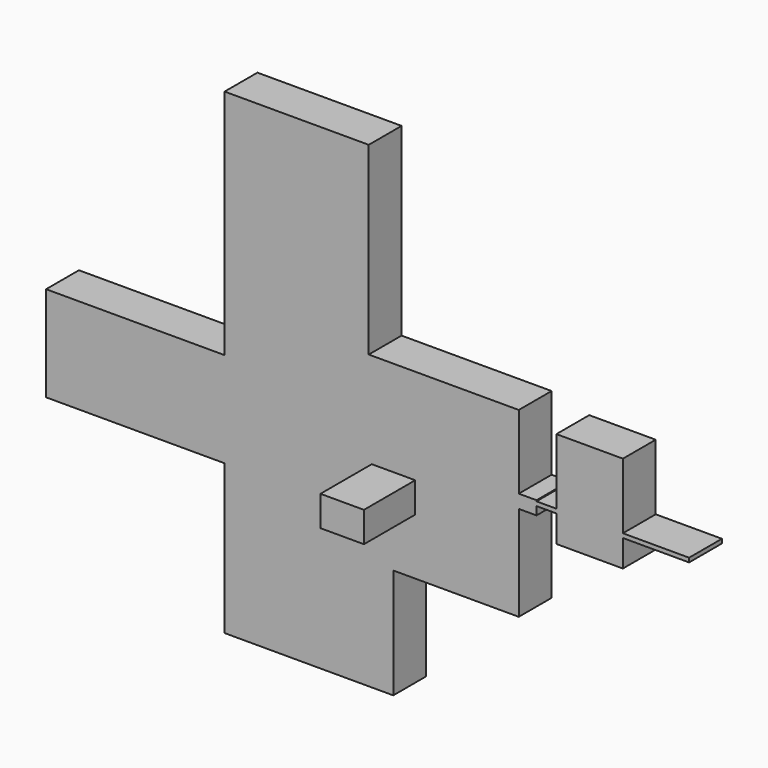
from build123d import *

# Parameters (mm, degrees)
F0_W     = 94.794575125
F0_H     = 66.0311877728
F1_DEPTH = 229.37163
F2_W     = 367.8625924513
F2_H     = 239.847317338
F2_W_2   = 389.3495500088
F2_H_2   = 207.6520100236
F2_W_3   = 314.4028186798
F2_H_3   = 402.6826024055
F2_W_4   = 43.3726906776
F2_H_4   = 9.1089755297
F2_W_5   = 145.0487077236
F2_H_5   = 58.66086483
F2_H_6   = 143.2274132967
F2_W_6   = 144.3722844124
F3_DEPTH = 89.50501


with BuildPart() as f1:
    # F0 (on Front) → F1 (new body)
    with BuildSketch(Plane.XZ):
        with Locations((14.3123473972, 155.8356285095)):
            Rectangle(F0_W, F0_H)
    extrude(amount=F1_DEPTH)

    # F2 (on Front) → F3 (join)
    with BuildSketch(Plane.XZ):
        with Locations((-170.1408275403, -119.923658669)):
            Rectangle(F2_W, F2_H)
        Polygon((-354.0721237659, 0), (13.7904686853, 0), (287.5355780125, 0), (287.5355780125, 207.2783261538), (287.5355780125, 236.5134656429), (287.5355780125, 397.2084522247), (-39.6693050861, 397.2084522247), (-354.0721237659, 397.2084522247), (-354.0721237659, 293.8325405121), (-354.0721237659, 86.1805304885), align=None)
        with Locations((-548.7468987703, 190.0065355003)):
            Rectangle(F2_W_2, F2_H_2)
        Polygon((287.5355780125, 236.5134656429), (287.5355780125, 207.2783261538), (326.2129127979, 207.2783261538), (326.2129127979, 225.2303659916), (326.2129127979, 234.3393415213), (326.2129127979, 236.5134656429), align=None)
        with Locations((-196.870714426, 598.5497534275)):
            Rectangle(F2_W_3, F2_H_3)
        with Locations((347.8992581367, 229.7848537564)):
            Rectangle(F2_W_4, F2_H_4)
        with Locations((442.1099573374, 229.7848537564)):
            Rectangle(F2_W_5, F2_H_4)
        with Locations((442.1099573374, 195.8999335766)):
            Rectangle(F2_W_5, F2_H_5)
        with Locations((442.1099573374, 305.9530481696)):
            Rectangle(F2_W_5, F2_H_6)
        with Locations((586.8204534054, 229.7848537564)):
            Rectangle(F2_W_6, F2_H_4)
    extrude(amount=F3_DEPTH)


solid = f1.part
